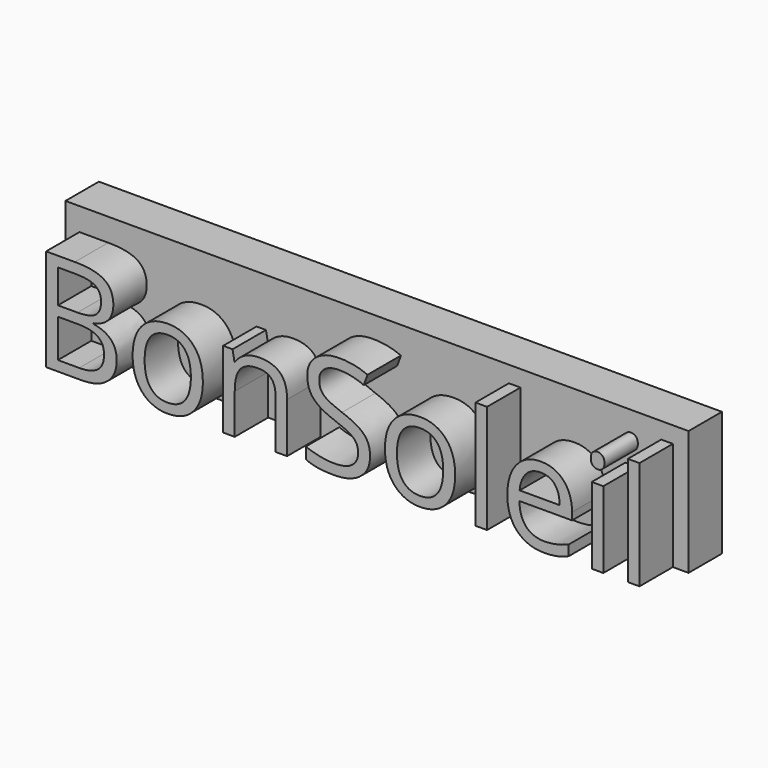
from build123d import *

# Parameters (mm, degrees)
F0_TEXT_SIZE = 17.1088133061
F1_DEPTH     = 5
F2_W         = 74.637286365
F2_H         = 14.9564975873
F3_DEPTH     = 5


# Not quite as in the source:
# - Text() gives the source's letters only with a copy of the font that has no kerning and outlines rounded to 1/6400 em; it was checked with that copy


with BuildPart() as f1:
    # F0 (on Front) → F1 (new body)
    with BuildSketch(Plane.XZ):
        with Locations((0, 0)):
            Text('BonSoleil', F0_TEXT_SIZE, font='Open Sans', text_align=(TextAlign.LEFT, TextAlign.BOTTOM))
    extrude(amount=F1_DEPTH)


with BuildPart() as f3:
    # F2 (on Front) → F3 (new body)
    with BuildSketch(Plane.XZ):
        with Locations((37.3186431825, 7.4782487936)):
            Rectangle(F2_W, F2_H)
    extrude(amount=-F3_DEPTH)


solid = Compound([f1.part, f3.part])
